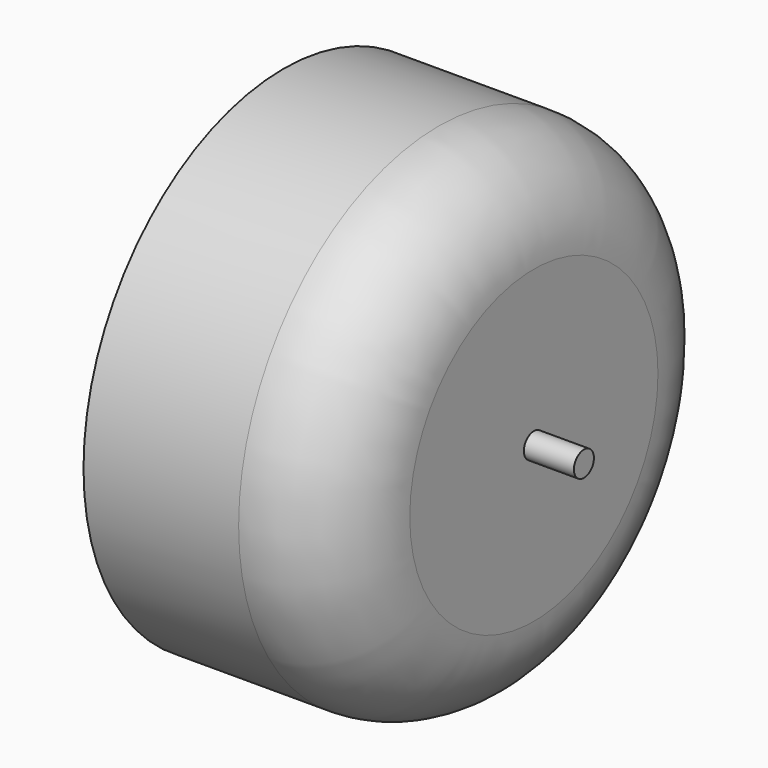
from build123d import *

# Parameters (mm, degrees)
F0_R     = 127
F1_DEPTH = 127
F2_R     = 114.3
F3_DEPTH = 101.6
F4_R     = 48.26
F6_R     = 6.35
F7_DEPTH = 25.4
F8_R     = 19.05
F9_DEPTH = 76.2


# Not quite as in the source:
# - a fillet or chamfer that OpenCascade refuses, or shapes differently, is made with other operations: its cross-section is extruded or revolved along the edge and cut away or added


with BuildPart() as f1:
    # F0 (on Right) → F1 (new body)
    with BuildSketch(Plane.YZ):
        Circle(F0_R)
    extrude(amount=F1_DEPTH)

    # F2 (on Right) → F3 (cut)
    with BuildSketch(Plane.YZ):
        Circle(F2_R)
    extrude(amount=F3_DEPTH, mode=Mode.SUBTRACT)

    # F4
    f4_edges = [f1.edges().sort_by_distance(p)[0] for p in [
        (127, -127, 0),
    ]]
    fillet(f4_edges, radius=F4_R)

    # F5: fillet of radius 63.5 on 3 edges, made by hand

    # F5_s1 → F5_t2 (revolve)
    with BuildSketch(Plane.XY):
        with BuildLine():
            ThreePointArc((38.1, 114.3), (83.0012806053, 95.7012806053), (101.6, 50.8))
            Line((101.6, 50.8), (101.6, 114.3))
            Line((101.6, 114.3), (38.1, 114.3))
        make_face()
    revolve(axis=Axis((101.6, 0, 0), (1, 0, 0)))

    # F5_s3 → F5_t4 (revolve, cut)
    with BuildSketch(Plane.XY):
        with BuildLine():
            ThreePointArc((0, 127), (18.0195368579, 117.5586105738), (38.1, 114.3))
            Line((38.1, 114.3), (38.1, 107.95))
            Line((38.1, 107.95), (0, 107.95))
            Line((0, 107.95), (-6.35, 114.3))
            ThreePointArc((-6.35, 114.3), (-6.35, 120.65), (-3.81, 121.92))
            Line((-3.81, 121.92), (0, 127))
        make_face()
    revolve(axis=Axis((0, 0, 0), (1, 0, 0)), mode=Mode.SUBTRACT)

    # F6 (on face) → F7 (join)
    with BuildSketch(Plane.YZ.offset(127)):
        Circle(F6_R)
    extrude(amount=F7_DEPTH)

    # F8 (on face) → F9 (join)
    with BuildSketch(Plane(origin=(101.6, 0, 0), x_dir=(0, -1, 0), z_dir=(-1, 0, 0))):
        Circle(F8_R)
    extrude(amount=F9_DEPTH)


solid = f1.part
